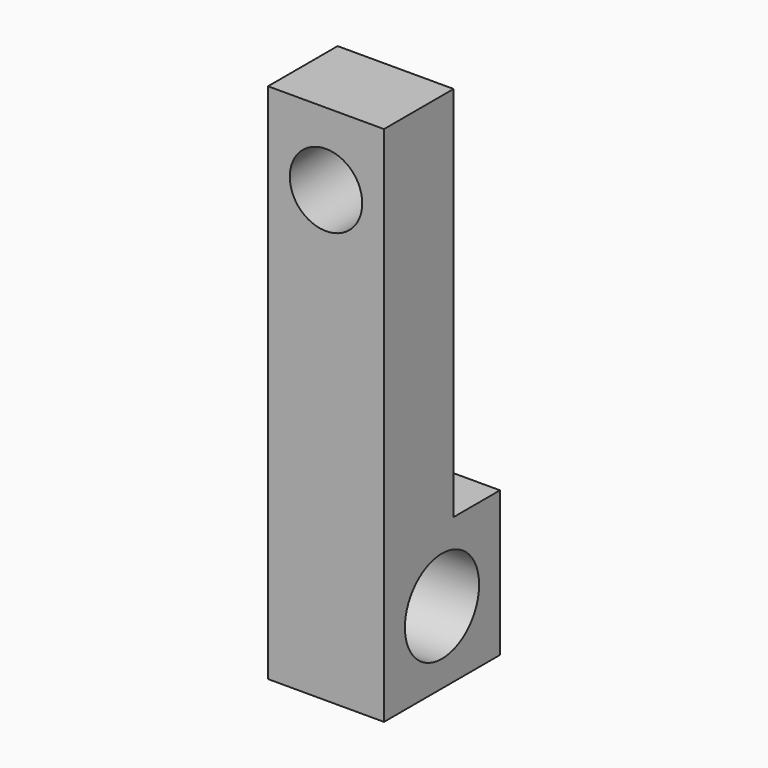
from build123d import *

# Parameters (mm, degrees)
F0_R     = 1.6
F0_W     = 3
F0_H     = 13
F1_DEPTH = 4
F2_R     = 1.25
F3_DEPTH = 25


# Not quite as in the source:
# - a feature names something its author has since deleted; it is built from what else it names


with BuildPart() as f1:
    # F0 (on Right) → F1 (new body)
    with BuildSketch(Plane.YZ):
        Polygon((-2.5, -2.5), (2.5, -2.5), (2.5, 2.5), (0.5, 2.5), (-2.5, 2.5), align=None)
        Circle(F0_R, mode=Mode.SUBTRACT)
        with Locations((-1, 9)):
            Rectangle(F0_W, F0_H)
    extrude(amount=-F1_DEPTH)

    # F2 (on face) → F3 (cut)
    with BuildSketch(Plane.XZ.offset(2.5)):
        with Locations((-2, 13)):
            Circle(F2_R)
    extrude(amount=-F3_DEPTH, mode=Mode.SUBTRACT)


solid = f1.part
